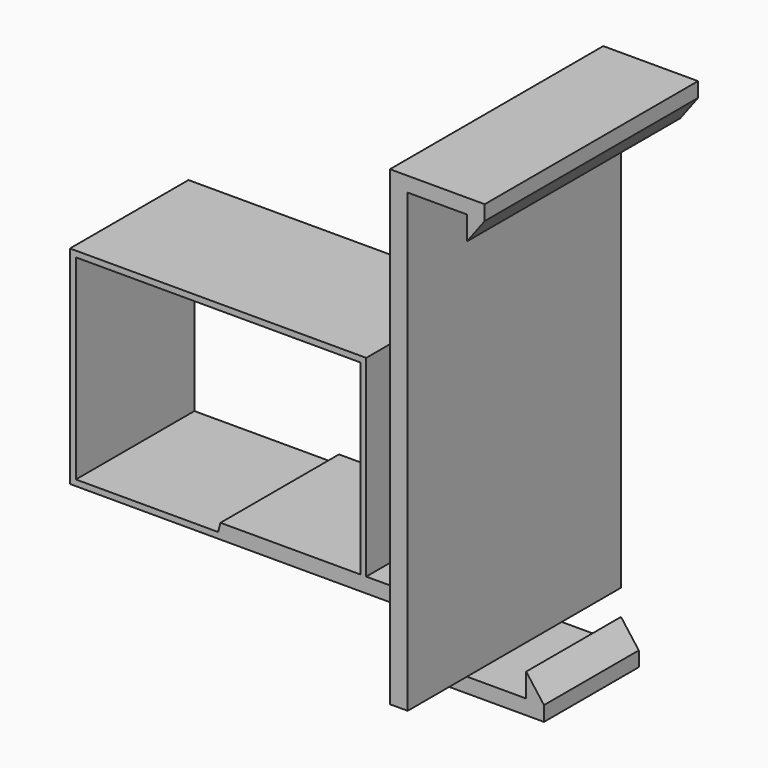
from build123d import *

# Parameters (mm, degrees)
F1_DEPTH = 22.5
F2_DEPTH = 10
F0_W     = 12
F0_H     = 2.5
F3_DEPTH = 12.5
F4_DEPTH = 12.5
F5_DEPTH = 12.5


# Not quite as in the source:
# - a feature names something its author has since deleted; it is built from what else it names


with BuildPart() as f1:
    # F0 (on Front) → F1 (new body, symmetric)
    with BuildSketch(Plane.XZ):
        Polygon((8, 38.5), (8, 41), (-8, 41), (-8, 8), (-8, -27.5), (-8, -30), (-8, -38.5), (-5, -38.5), (-5, 38.5), (5, 38.5), (5, 34.5), align=None)
    extrude(amount=F1_DEPTH, both=True)

    # F0 (on Front) → F2 (join, symmetric)
    with BuildSketch(Plane.XZ):
        Polygon((-5, -38.5), (-8, -38.5), (-8, -41), (8, -41), (8, -38.5), (5, -34.5), (5, -38.5), align=None)
    extrude(amount=F2_DEPTH, both=True)

    # F0 (on Front) → F3 (join, symmetric)
    with BuildSketch(Plane.XZ):
        with Locations((-14, -28.75)):
            Rectangle(F0_W, F0_H)
    extrude(amount=F3_DEPTH, both=True)

    # F0 (on Front) → F4 (join, symmetric)
    with BuildSketch(Plane.XZ):
        Polygon((-20, -30), (-20, -27.5), (-20, 5), (-70, 5), (-70, -30), (-44.4338369071, -30), align=None)
        Polygon((-21, 4), (-21, -27.5), (-21, -29), (-45, -29), (-69, -29), (-69, 4), align=None, mode=Mode.SUBTRACT)
    extrude(amount=F4_DEPTH, both=True)

    # F0 (on Front) → F5 (join, symmetric)
    with BuildSketch(Plane.XZ):
        Polygon((-21, -29), (-21, -27.5), (-44.5986762643, -27.5), (-45, -29), align=None)
    extrude(amount=F5_DEPTH, both=True)


solid = f1.part
